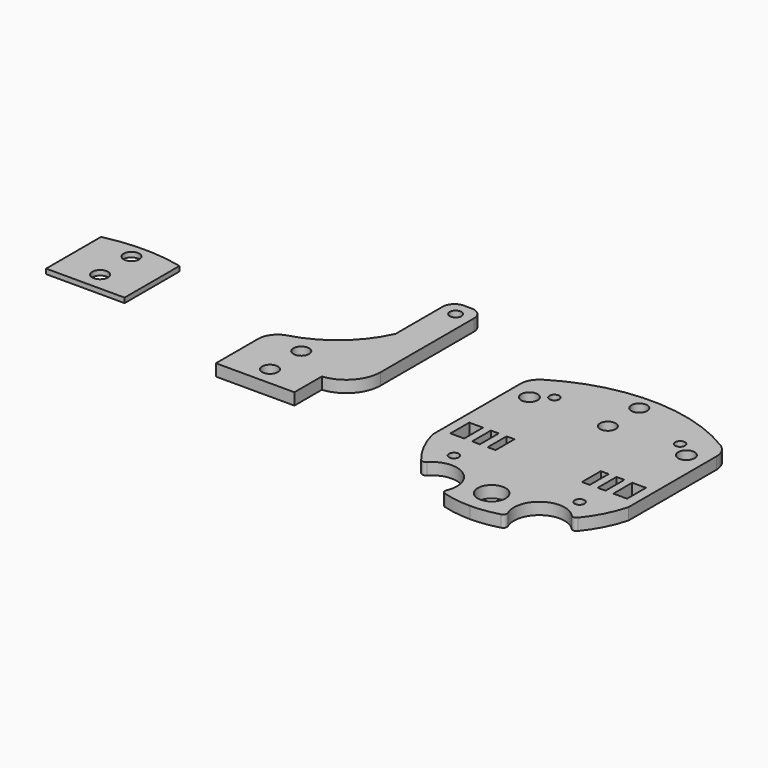
from build123d import *

# Parameters (mm, degrees)
F0_R     = 1.25
F0_R_2   = 3.555
F0_W     = 3.5
F0_H     = 6
F0_W_2   = 2
F0_R_3   = 2.1
F0_R_4   = 2
F1_DEPTH = 3
F0_R_5   = 1.5
F2_DEPTH = 3
F4_R     = 2.1
F4_R_2   = 2.25
F5_DEPTH = 25
F6_DEPTH = 1.25


# Not quite as in the source:
# - a feature names something its author has since deleted; it is built from what else it names


with BuildPart() as f1:
    # F0 (on Top) → F1 (new body)
    with BuildSketch(Plane.XY):
        with BuildLine():
            Line((25, 14.3136761677), (-25, 14.3136761677))
            Line((-25, 14.3136761677), (-25, -5.6028405869))
            ThreePointArc((-25, -5.6028405869), (-23.0117824833, -10.8325706042), (-19.9442440013, -15.5115974911))
            ThreePointArc((-19.9442440013, -15.5115974911), (-19.2052482882, -15.8754446325), (-18.443850882, -15.5611622815))
            ThreePointArc((-18.443850882, -15.5611622815), (-10.1760612052, -14.5858281895), (-7.7862204272, -22.5605560084))
            ThreePointArc((-7.7862204272, -22.5605560084), (-7.7721201862, -23.38414607), (-7.1446119827, -23.9177497252))
            ThreePointArc((-7.1446119827, -23.9177497252), (-3.6076561704, -24.6722072912), (0, -24.9253467642))
            ThreePointArc((0, -24.9253467642), (3.6076561704, -24.6722072912), (7.1446119827, -23.9177497252))
            ThreePointArc((7.1446119827, -23.9177497252), (7.7721201862, -23.38414607), (7.7862204272, -22.5605560084))
            ThreePointArc((7.7862204272, -22.5605560084), (10.1760612052, -14.5858281895), (18.443850882, -15.5611622815))
            ThreePointArc((18.443850882, -15.5611622815), (19.2052482882, -15.8754446325), (19.9442440013, -15.5115974911))
            ThreePointArc((19.9442440013, -15.5115974911), (23.0117824833, -10.8325706042), (25, -5.6028405869))
            Line((25, -5.6028405869), (25, 14.3136761677))
        make_face()
        with Locations((-16, -10)):
            Circle(F0_R, mode=Mode.SUBTRACT)
        with Locations((0, -18)):
            Circle(F0_R_2, mode=Mode.SUBTRACT)
        with Locations((16, -10)):
            Circle(F0_R, mode=Mode.SUBTRACT)
        with Locations((-20.75, 0)):
            Rectangle(F0_W, F0_H, mode=Mode.SUBTRACT)
        with Locations((-16, 0)):
            Rectangle(F0_W_2, F0_H, mode=Mode.SUBTRACT)
        with Locations((-12, 0)):
            Rectangle(F0_W_2, F0_H, mode=Mode.SUBTRACT)
        with Locations((12, 0)):
            Rectangle(F0_W_2, F0_H, mode=Mode.SUBTRACT)
        with Locations((16, 0)):
            Rectangle(F0_W_2, F0_H, mode=Mode.SUBTRACT)
        with Locations((20.75, 0)):
            Rectangle(F0_W, F0_H, mode=Mode.SUBTRACT)
        with BuildLine():
            ThreePointArc((-22.6164226719, 26.5744662824), (-24.3636059263, 24.7547708647), (-25, 22.3136761677))
            Line((-25, 22.3136761677), (-25, 14.3136761677))
            Line((-25, 14.3136761677), (25, 14.3136761677))
            Line((25, 14.3136761677), (25, 22.3136761677))
            ThreePointArc((25, 22.3136761677), (24.3636059263, 24.7547708647), (22.6164226719, 26.5744662824))
            ThreePointArc((22.6164226719, 26.5744662824), (0, 32.964214922), (-22.6164226719, 26.5744662824))
        make_face()
        with Locations((-20, 19)):
            Circle(F0_R_3, mode=Mode.SUBTRACT)
        with Locations((-16, 22)):
            Circle(F0_R, mode=Mode.SUBTRACT)
        with Locations((0, 19)):
            Circle(F0_R_4, mode=Mode.SUBTRACT)
        with Locations((20, 19)):
            Circle(F0_R_3, mode=Mode.SUBTRACT)
        with Locations((16, 22)):
            Circle(F0_R, mode=Mode.SUBTRACT)
        with Locations((0, 29)):
            Circle(F0_R_4, mode=Mode.SUBTRACT)
    extrude(amount=F1_DEPTH)


with BuildPart() as f1b:
    # F0 (on Top) → F1, piece 2 (new body)
    with BuildSketch(Plane.XY):
        with BuildLine():
            Line((-77.8149985122, 4.86868793), (-77.8149985122, -8.5344709849))
            Line((-77.8149985122, -8.5344709849), (-57.8149985122, -8.5344709849))
            Line((-57.8149985122, -8.5344709849), (-57.8149985122, 0.2044082856))
            ThreePointArc((-57.8149985122, 0.2044082856), (-52.1170226198, 3.0194368328), (-49.8149985122, 8.9432869322))
            Line((-49.8149985122, 8.9432869322), (-49.8149985122, 38.6662318432))
            ThreePointArc((-49.8149985122, 38.6662318432), (-50.6936781686, 40.7875521867), (-52.8149985122, 41.6662318432))
            Line((-52.8149985122, 41.6662318432), (-54.8149985122, 41.6662318432))
            ThreePointArc((-54.8149985122, 41.6662318432), (-56.9363188557, 40.7875521867), (-57.8149985122, 38.6662318432))
            Line((-57.8149985122, 38.6662318432), (-57.8149985122, 23.6662318432))
            ThreePointArc((-57.8149985122, 23.6662318432), (-64.445474594, 14.8702366754), (-74.1630322412, 9.6835404787))
            ThreePointArc((-74.1630322412, 9.6835404787), (-76.798725953, 7.8902629626), (-77.8149985122, 4.86868793))
        make_face()
        with Locations((-67.7919896514, -3.8481471525)):
            Circle(F0_R_4, mode=Mode.SUBTRACT)
        with Locations((-67.8149985122, 6.1518528475)):
            Circle(F0_R_4, mode=Mode.SUBTRACT)
        with Locations((-53.8149985122, 37.8072073483)):
            Circle(F0_R_5, mode=Mode.SUBTRACT)
    extrude(amount=F1_DEPTH)


with BuildPart() as f2:
    # F0 (on Top) → F2 (new body)
    with BuildSketch(Plane.XY):
        with BuildLine():
            ThreePointArc((-22.6164226719, 26.5744662824), (-24.3636059263, 24.7547708647), (-25, 22.3136761677))
            Line((-25, 22.3136761677), (-25, 14.3136761677))
            Line((-25, 14.3136761677), (25, 14.3136761677))
            Line((25, 14.3136761677), (25, 22.3136761677))
            ThreePointArc((25, 22.3136761677), (24.3636059263, 24.7547708647), (22.6164226719, 26.5744662824))
            ThreePointArc((22.6164226719, 26.5744662824), (0, 32.964214922), (-22.6164226719, 26.5744662824))
        make_face()
        with Locations((-20, 19)):
            Circle(F0_R_3, mode=Mode.SUBTRACT)
        with Locations((-16, 22)):
            Circle(F0_R, mode=Mode.SUBTRACT)
        with Locations((0, 19)):
            Circle(F0_R_4, mode=Mode.SUBTRACT)
        with Locations((20, 19)):
            Circle(F0_R_3, mode=Mode.SUBTRACT)
        with Locations((16, 22)):
            Circle(F0_R, mode=Mode.SUBTRACT)
        with Locations((0, 29)):
            Circle(F0_R_4, mode=Mode.SUBTRACT)
        with Locations((-16, 22)):
            Circle(F0_R)
        with Locations((16, 22)):
            Circle(F0_R)
    extrude(amount=F2_DEPTH)


with BuildPart() as f2_1:
    # F3: moved
    add(f2.part.moved(Location((55.75, 0, 0))))

    # F4 (on face) → F5 (cut)
    with BuildSketch(Plane.XY.offset(3)):
        with BuildLine():
            Line((30.75, 14.3136761677), (45.75, 14.3136761677))
            Line((45.75, 14.3136761677), (45.75, 25.7562933257))
            ThreePointArc((45.75, 25.7562933257), (46.2050390496, 27.8403590538), (47.4873319836, 29.5450922667))
            ThreePointArc((47.4873319836, 29.5450922667), (51.3440284338, 31.9183440188), (55.75, 32.964214922))
            ThreePointArc((55.75, 32.964214922), (43.9991334133, 31.3361124445), (33.1335773281, 26.5744662824))
            ThreePointArc((33.1335773281, 26.5744662824), (31.3863940737, 24.7547708647), (30.75, 22.3136761677))
            Line((30.75, 22.3136761677), (30.75, 14.3136761677))
        make_face()
        with Locations((35.75, 19)):
            Circle(F4_R, mode=Mode.SUBTRACT)
        with Locations((42.75, 19)):
            Circle(F4_R_2, mode=Mode.SUBTRACT)
        with BuildLine():
            ThreePointArc((58.8838195988, 32.8504511649), (60.9470746388, 32.3880346997), (62.9193889887, 31.6259149894))
            ThreePointArc((62.9193889887, 31.6259149894), (70.6461883393, 24.5054009937), (73.2023363863, 14.3136761677))
            Line((73.2023363863, 14.3136761677), (80.75, 14.3136761677))
            Line((80.75, 14.3136761677), (80.75, 22.3136761677))
            ThreePointArc((80.75, 22.3136761677), (80.1136059263, 24.7547708647), (78.3664226719, 26.5744662824))
            ThreePointArc((78.3664226719, 26.5744662824), (69.0020089349, 30.8824353153), (58.8838195988, 32.8504511649))
        make_face()
        with Locations((75.75, 19)):
            Circle(F4_R, mode=Mode.SUBTRACT)
        with Locations((42.75, 19)):
            Circle(F4_R_2)
        with Locations((68.75, 19)):
            Circle(F4_R_2)
    extrude(amount=-F5_DEPTH, mode=Mode.SUBTRACT)


with BuildPart() as f6:
    # F0 (on Top) → F6 (new body)
    with BuildSketch(Plane.XY):
        with BuildLine():
            Line((-111.7582723053, 4.8228372639), (-111.7582723053, 22.3005958048))
            ThreePointArc((-111.7582723053, 22.3005958048), (-121.7582723053, 23.4733760182), (-131.7582723053, 22.3005958048))
            Line((-131.7582723053, 22.3005958048), (-131.7582723053, 4.8228372639))
            Line((-131.7582723053, 4.8228372639), (-111.7582723053, 4.8228372639))
        make_face()
        with Locations((-121.7352634446, 9.5091610962)):
            Circle(F0_R_4, mode=Mode.SUBTRACT)
        with Locations((-121.7582723053, 19.5091610962)):
            Circle(F0_R_4, mode=Mode.SUBTRACT)
    extrude(amount=F6_DEPTH)


solid = Compound([f1.part, f1b.part, f6.part])
